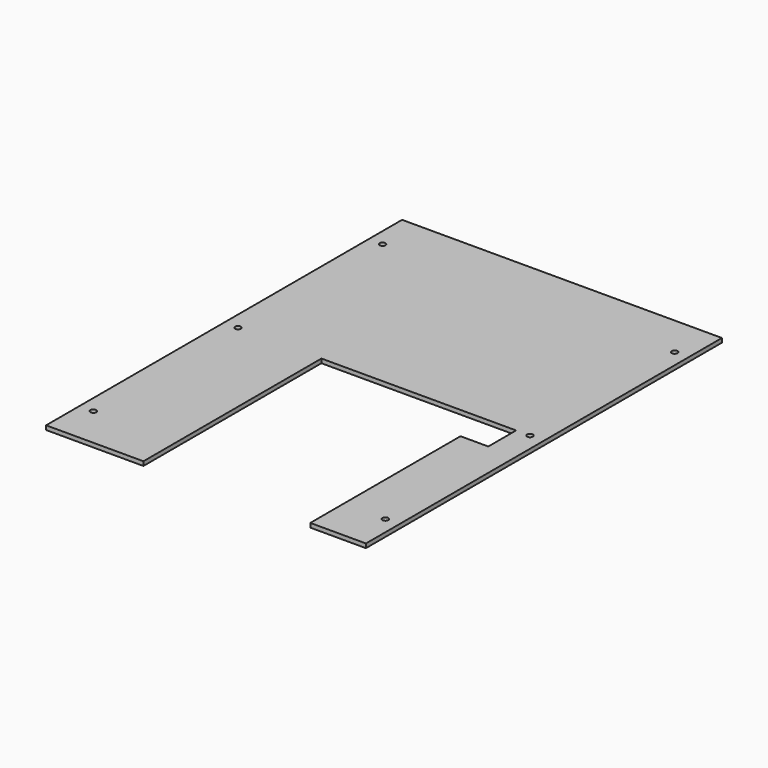
from build123d import *

# Parameters (mm, degrees)
F1_W     = 230
F1_H     = 320
F2_DEPTH = 3
F4_D     = 4.2
F4_DEPTH = 4
F4_TIP   = 1.2618073
F5_W     = 120
F5_H     = 160
F6_DEPTH = 25
F7_W     = 20
F7_H     = 25
F8_DEPTH = 3


# Not quite as in the source:
# - a pattern or mirror of a feature is missing from the dataset's text; its kind, count and spacing are read off the source's solid


with BuildPart() as f2:
    # F1 (on Top) → F2 (new body)
    with BuildSketch(Plane.XY):
        Rectangle(F1_W, F1_H)
    extrude(amount=F2_DEPTH)

    # F4
    with Locations(Plane.XY.offset(3)):
        with Locations((-105, 130), (-105, 0), (-105, -130)):
            f4 = Hole(F4_D / 2, depth=F4_DEPTH)
            with Locations((0, 0, -(F4_DEPTH + F4_TIP / 2))):  # 118° drill point
                Cone(0, F4_D / 2, F4_TIP, mode=Mode.SUBTRACT)

    # F4_copies: F4 across plane
    add(f4.mirror(Plane(origin=(0, 0, 0), x_dir=(0, 0, 1), z_dir=(1, 0, 0))), mode=Mode.SUBTRACT)

    # F5 (on face) → F6 (cut)
    with BuildSketch(Plane.XY.offset(3)):
        with Locations((15, -80)):
            Rectangle(F5_W, F5_H)
    extrude(amount=-F6_DEPTH, mode=Mode.SUBTRACT)

    # F7 (on face) → F8 (cut, through all)
    with BuildSketch(Plane.XY.offset(3)):
        with Locations((85, -12.5)):
            Rectangle(F7_W, F7_H)
    extrude(amount=-F8_DEPTH, mode=Mode.SUBTRACT)


solid = f2.part
